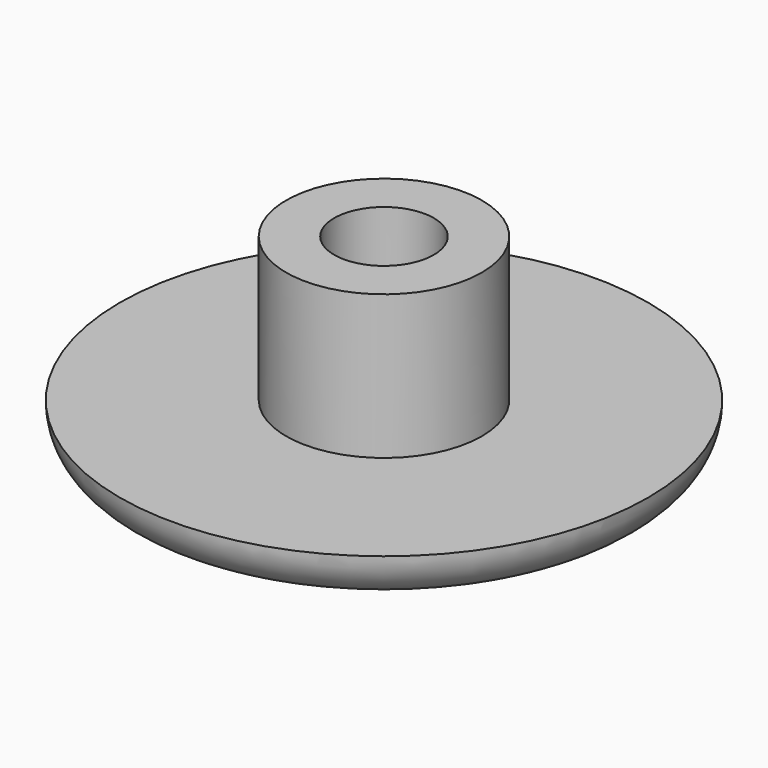
from build123d import *

# Parameters (mm, degrees)
F0_R     = 11
F1_DEPTH = 2
F3_R     = 4.075
F3_R_2   = 2.075
F4_DEPTH = 6
F5_R     = 1.99999
F6_R     = 2


# Not quite as in the source:
# - a fillet or chamfer is up to 0.001 mm smaller than in the source, because OpenCascade refuses the exact size
# - a feature names something its author has since deleted; it is built from what else it names


with BuildPart() as f1:
    # F0 (on Top) → F1 (new body)
    with BuildSketch(Plane.XY):
        with Locations((0, 21.965100023)):
            Circle(F0_R)
    extrude(amount=F1_DEPTH)

    # F3 (on face) → F4 (join)
    with BuildSketch(Plane.XY.offset(2)):
        with Locations((0, 21.965100023)):
            Circle(F3_R)
        with Locations((0, 21.965100023)):
            Circle(F3_R_2, mode=Mode.SUBTRACT)
    extrude(amount=F4_DEPTH)

    # F5 (radius 2 in the source; OpenCascade refuses exactly that, so slightly less here)
    f5_edges = [f1.edges().sort_by_distance(p)[0] for p in [
        (-11, 21.9651, 0),
    ]]
    fillet(f5_edges, radius=F5_R)

    # F6
    f6_edges = [f1.edges().sort_by_distance(p)[0] for p in [
        (-2.075, 21.9651, 2),
    ]]
    fillet(f6_edges, radius=F6_R)


solid = f1.part
